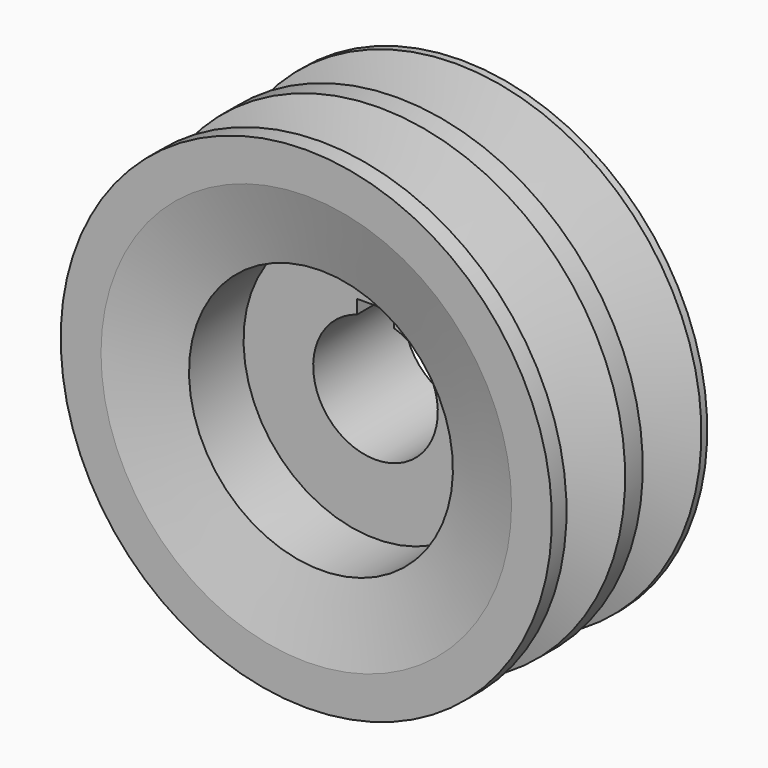
from build123d import *

# Parameters (mm, degrees)
F2_W     = 5
F2_H     = 3
F3_DEPTH = 27.301


# Not quite as in the source:
# - ends of sketch curves that miss each other by under 0.0002 mm in the source are joined


with BuildPart() as f1:
    # F0 (on Right) → F1 (revolve)
    with BuildSketch(Plane.YZ):
        Polygon((2.5, 33.5), (0, 33.5), (0, 28), (2.5, 18), (11.8, 18), (11.8, 8.5), (27.3, 8.5), (27.3, 13), (26.5, 13), (26.5, 33.5), (25.5, 33.5), (21.0595629684, 21.3), (19.940437, 21.3), (15.5, 33.5), (12.5, 33.5), (8.0595629684, 21.3), (6.940437, 21.3), align=None)
    revolve(axis=Axis((0, 13.65, 0), (0, 1, 0)))

    # F2 (on Front) → F3 (cut, through all)
    with BuildSketch(Plane.XZ):
        with Locations((0, 8.5)):
            Rectangle(F2_W, F2_H)
    extrude(amount=-F3_DEPTH, mode=Mode.SUBTRACT)


solid = f1.part
